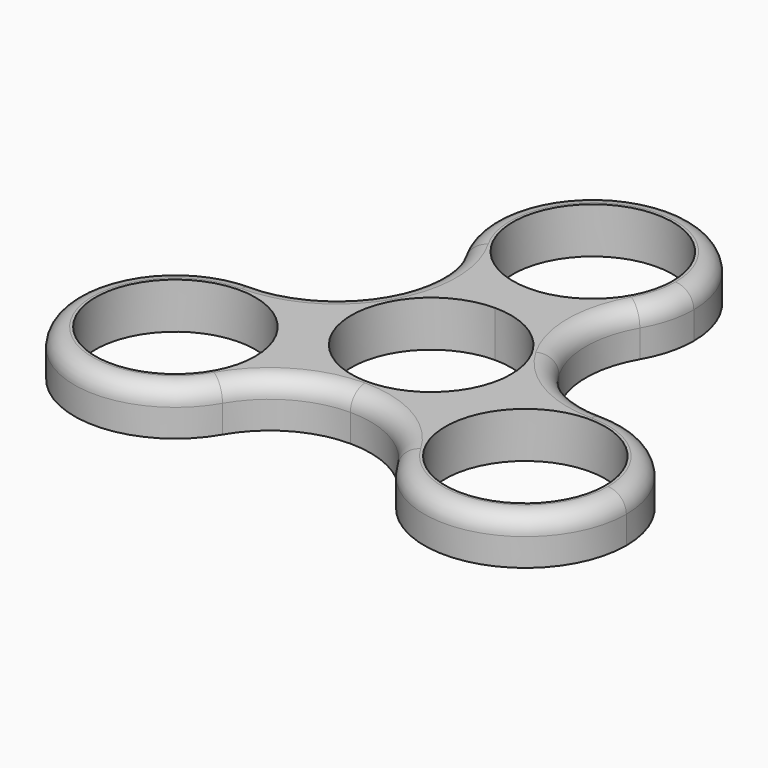
from build123d import *

# Parameters (mm, degrees)
F0_R     = 11.049
F1_DEPTH = 6.35
F2_R     = 2.54


# Not quite as in the source:
# - ends of sketch curves that miss each other by under 0.0002 mm in the source are joined


with BuildPart() as f1:
    # F0 (on Top) → F1 (new body)
    with BuildSketch(Plane.XY):
        with BuildLine():
            ThreePointArc((0, 11.049), (7.8128228253, 7.8128228253), (11.049, 0))
            ThreePointArc((11.049, 0), (-2.8596916293, -10.6725144547), (-9.5687146864, 5.5245))
            Line((-9.5687146864, 5.5245), (-12.0983748909, 6.985))
            ThreePointArc((-12.0983748909, 6.985), (-13.97, 3.443e-07), (-12.0983754224, -6.9849990793))
            ThreePointArc((-12.0983754224, -6.9849990793), (-6.9850004566, -12.0983746273), (8.7e-09, -13.97))
            ThreePointArc((8.7e-09, -13.97), (6.9850004798, -12.0983746139), (12.0983754405, -6.984999048))
            ThreePointArc((12.0983754405, -6.984999048), (13.4939839355, -3.6157015292), (13.97, 0))
            ThreePointArc((13.97, 0), (13.4939839355, 3.6157015292), (12.0983754405, 6.984999048))
            ThreePointArc((12.0983754405, 6.984999048), (6.9850004648, 12.0983746225), (-2.58e-08, 13.97))
            Line((-2.58e-08, 13.97), (0, 11.049))
        make_face()
        with BuildLine():
            ThreePointArc((-9.5687146864, 5.5245), (-5.5245, 9.5687146864), (0, 11.049))
            Line((0, 11.049), (0, 13.97))
            ThreePointArc((0, 13.97), (-6.9850001734, 12.0983747908), (-12.0983750781, 6.9849996757))
            Line((-12.0983750781, 6.9849996757), (-9.5687146864, 5.5245))
        make_face()
        with BuildLine():
            ThreePointArc((-12.0983750781, 6.9849996757), (-6.9850001734, 12.0983747908), (-2.58e-08, 13.97))
            ThreePointArc((-2.58e-08, 13.97), (-6.9850000112, 15.8416251156), (-12.0983748909, 20.955))
            ThreePointArc((-12.0983748909, 20.955), (-10.2267497817, 13.9699998127), (-12.0983750781, 6.9849996757))
        make_face()
        with BuildLine():
            ThreePointArc((-12.0983748909, 20.955), (-6.9850000112, 15.8416251156), (-2.58e-08, 13.97))
            ThreePointArc((-2.58e-08, 13.97), (6.9849999888, 15.8416251027), (12.0983748909, 20.955))
            ThreePointArc((12.0983748909, 20.955), (13.4939837933, 24.3242979399), (13.97, 27.94))
            ThreePointArc((13.97, 27.94), (-3.6157020601, 41.4339837933), (-12.0983748909, 20.955))
        make_face()
        with BuildLine():
            ThreePointArc((11.049, 27.94), (7.8128228253, 20.1271771747), (0, 16.891))
            ThreePointArc((0, 16.891), (-7.8128228253, 35.7528228253), (11.049, 27.94))
        make_face(mode=Mode.SUBTRACT)
        with BuildLine():
            ThreePointArc((12.0983748909, 20.955), (6.9849999888, 15.8416251027), (-2.58e-08, 13.97))
            ThreePointArc((-2.58e-08, 13.97), (6.9850004648, 12.0983746225), (12.0983754405, 6.984999048))
            ThreePointArc((12.0983754405, 6.984999048), (10.2267497817, 13.9699994504), (12.0983748909, 20.955))
        make_face()
        with BuildLine():
            ThreePointArc((-12.0983754224, -6.9849990793), (-13.97, 3.443e-07), (-12.0983750781, 6.9849996757))
            ThreePointArc((-12.0983750781, 6.9849996757), (-17.2117499439, 1.8716250155), (-24.1967497817, 0))
            ThreePointArc((-24.1967497817, 0), (-17.2117502421, -1.8716248433), (-12.0983754224, -6.9849990793))
        make_face()
        with BuildLine():
            ThreePointArc((24.1967497817, 0), (17.2117502577, 1.8716248343), (12.0983754405, 6.984999048))
            ThreePointArc((12.0983754405, 6.984999048), (13.4939839355, 3.6157015292), (13.97, 0))
            ThreePointArc((13.97, 0), (13.4939839355, -3.6157015292), (12.0983754405, -6.984999048))
            ThreePointArc((12.0983754405, -6.984999048), (17.2117502577, -1.8716248343), (24.1967497817, 0))
        make_face()
        with BuildLine():
            ThreePointArc((8.7e-09, -13.97), (-6.9850004566, -12.0983746273), (-12.0983754224, -6.9849990793))
            ThreePointArc((-12.0983754224, -6.9849990793), (-10.7027661261, -10.3542974265), (-10.2267497817, -13.97))
            ThreePointArc((-10.2267497817, -13.97), (-10.7027659885, -17.5857020601), (-12.0983748909, -20.955))
            ThreePointArc((-12.0983748909, -20.955), (-6.9849999962, -15.841625107), (8.7e-09, -13.97))
        make_face()
        with BuildLine():
            ThreePointArc((-10.2267497817, -13.97), (-10.7027661261, -10.3542974265), (-12.0983754224, -6.9849990793))
            ThreePointArc((-12.0983754224, -6.9849990793), (-17.2117502421, -1.8716248433), (-24.1967497817, 0))
            ThreePointArc((-24.1967497817, 0), (-36.2951246726, -20.955), (-12.0983748909, -20.955))
            ThreePointArc((-12.0983748909, -20.955), (-10.7027659885, -17.5857020601), (-10.2267497817, -13.97))
        make_face()
        with Locations((-24.1967497817, -13.97)):
            Circle(F0_R, mode=Mode.SUBTRACT)
        with BuildLine():
            ThreePointArc((38.1667497817, -13.97), (34.0750315149, -4.0917182668), (24.1967497817, 0))
            ThreePointArc((24.1967497817, 0), (17.2117502577, -1.8716248343), (12.0983754405, -6.984999048))
            ThreePointArc((12.0983754405, -6.984999048), (10.2267497817, -13.9699994504), (12.0983748909, -20.955))
            ThreePointArc((12.0983748909, -20.955), (27.8124518418, -27.4639837933), (38.1667497817, -13.97))
        make_face()
        with Locations((24.1967497817, -13.97)):
            Circle(F0_R, mode=Mode.SUBTRACT)
        with BuildLine():
            ThreePointArc((12.0983754405, -6.984999048), (6.9850004798, -12.0983746139), (8.7e-09, -13.97))
            ThreePointArc((8.7e-09, -13.97), (6.9850000038, -15.8416251113), (12.0983748909, -20.955))
            ThreePointArc((12.0983748909, -20.955), (10.2267497817, -13.9699994504), (12.0983754405, -6.984999048))
        make_face()
    extrude(amount=F1_DEPTH)

    # F2
    f2_edges = [f1.edges().sort_by_distance(p)[0] for p in [
        (0, -13.97, 6.35),
        (36.295125, -20.955, 6.35),
        (12.098375, 6.985, 6.35),
        (0, 41.91, 6.35),
        (-12.098375, 6.985, 6.35),
        (-36.295125, -20.955, 6.35),
    ]]
    fillet(f2_edges, radius=F2_R)


solid = f1.part
